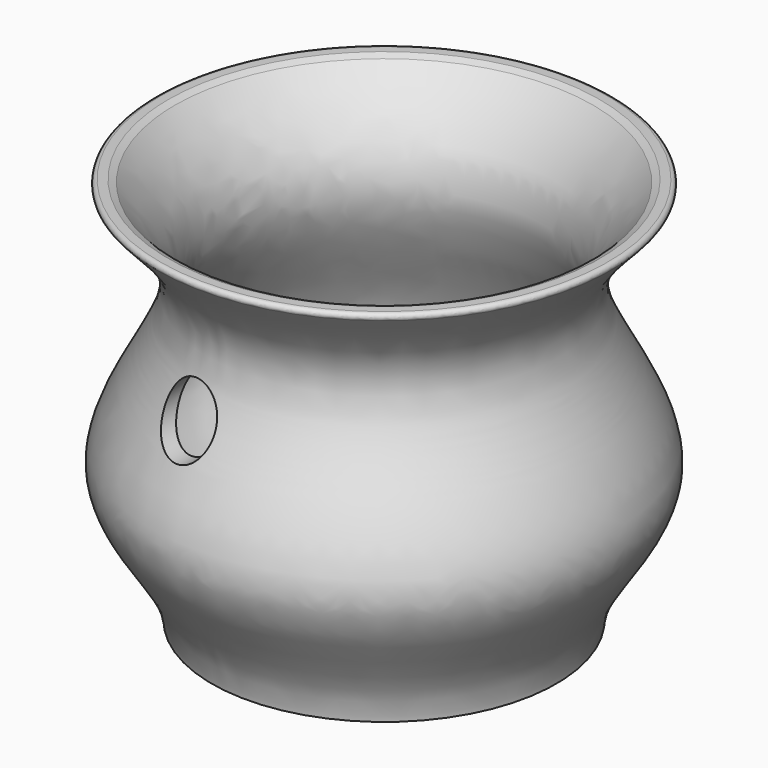
from build123d import *

# Parameters (mm, degrees)
F2_T     = -4
F3_R     = 1
F4_SIZE  = 1
F6_R     = 7.8874463413
F7_DEPTH = 50


with BuildPart() as f1:
    # F0 (on Front) → F1 (revolve)
    with BuildSketch(Plane.XZ):
        with BuildLine():
            Line((-44.3753963917, 0), (0, 0))
            Line((0, 0), (0, 100))
            Line((0, 100), (-60, 100))
            add(Edge.make_bspline(
                [(-60, 100), (-52.6541621731, 91.9218958662), (-33.8978285257, 75.9595428014), (-74.5456569157, 33.3173476275), (-45, 12.8346048295), (-44.3753963917, 0)],
                knots=[0, 0, 0, 0, 0.297877493, 0.6584550367, 1, 1, 1, 1], degree=3))
        make_face()
    revolve(axis=Axis((0, 0, 50), (0, 0, 1)))

    # F2
    f2_openings = [f1.faces().sort_by_distance(p)[0] for p in [
        (0, 0, 100),
    ]]
    offset(amount=F2_T, openings=f2_openings)

    # F3
    f3_edges = [f1.edges().sort_by_distance(p)[0] for p in [
        (60, 0, 100),
    ]]
    fillet(f3_edges, radius=F3_R)

    # F4
    f4_edges = [f1.edges().sort_by_distance(p)[0] for p in [
        (54.539195, 0, 100),
    ]]
    chamfer(f4_edges, length=F4_SIZE)

    # F6 (on offset) → F7 (cut)
    with BuildSketch(Plane.XZ.offset(80)):
        with Locations((-11.6351954639, 61.2611956894)):
            Circle(F6_R)
    extrude(amount=-F7_DEPTH, mode=Mode.SUBTRACT)


solid = f1.part
